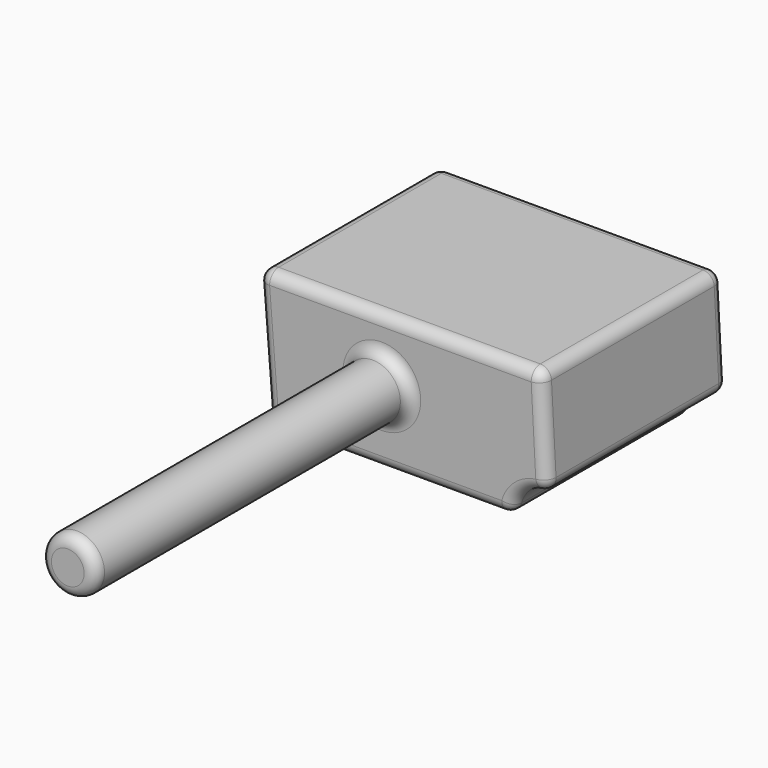
from build123d import *

# Parameters (mm, degrees)
F1_DEPTH = 50.8
F2_R     = 6.217599599
F3_DEPTH = 88.2316216
F4_R     = 2.54


# Not quite as in the source:
# - an extrude ends at something that could not be found from the text; its depth is read off the source's solid


with BuildPart() as f1:
    # F0 (on Front) → F1 (new body)
    with BuildSketch(Plane.XZ):
        with BuildLine():
            Line((1.2967513424, -23.9979514112), (0, 0))
            Line((0, 0), (-63.9691352844, 0))
            Line((-63.9691352844, 0), (-61.5289509296, -30.7046994567))
            Line((-61.5289509296, -30.7046994567), (-6.8309613811, -30.7046994567))
            ThreePointArc((-6.8309613811, -30.7046994567), (-4.3476416049, -25.4359191552), (1.2967513424, -23.9979514112))
        make_face()
    extrude(amount=F1_DEPTH)

    # F2 (on face) → F3 (join, through all)
    with BuildSketch(Plane.XZ.offset(50.8)):
        with Locations((-36.0038354993, -14.3174901605)):
            Circle(F2_R)
    extrude(amount=F3_DEPTH)

    # F4
    f4_edges = [f1.edges().sort_by_distance(p)[0] for p in [
        (-42.221435, -139.031622, -14.31749),
        (-61.528951, -25.4, -30.704699),
        (-63.969135, -25.4, 0),
        (1.296751, -25.4, -23.997951),
        (-6.830961, -25.4, -30.704699),
        (0, -25.4, 0),
        (-31.984568, 0, 0),
        (-62.749043, 0, -15.35235),
        (-34.179956, 0, -30.704699),
        (-4.347642, 0, -25.435919),
        (0.648376, 0, -11.998976),
        (-31.984568, -50.8, 0),
        (0.648376, -50.8, -11.998976),
        (-4.347642, -50.8, -25.435919),
        (-34.179956, -50.8, -30.704699),
        (-62.749043, -50.8, -15.35235),
        (-42.221435, -50.8, -14.31749),
    ]]
    fillet(f4_edges, radius=F4_R)


solid = f1.part
